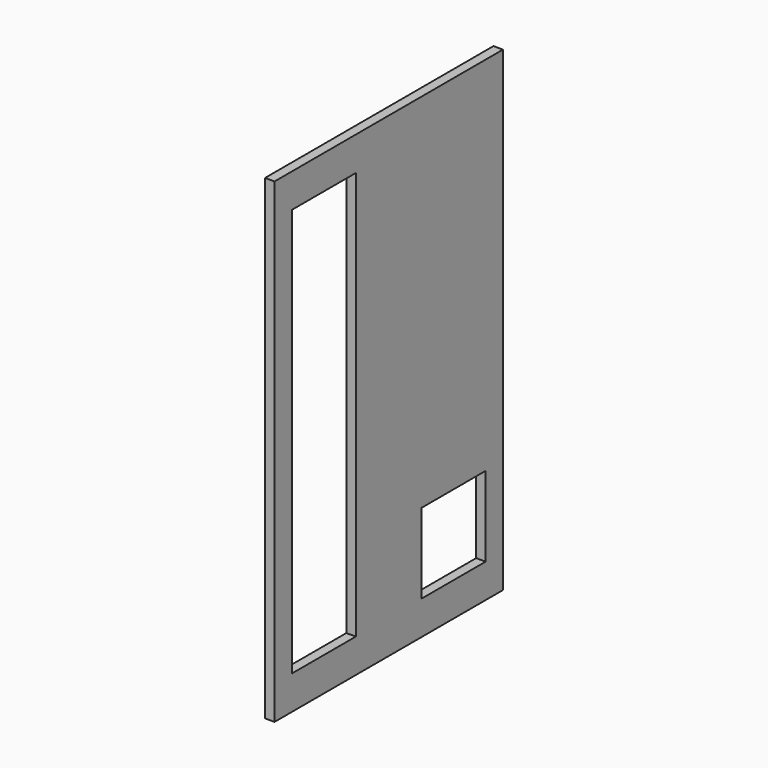
from build123d import *

# Parameters (mm, degrees)
F0_W     = 13.9900064
F0_H     = 3.81
F0_W_2   = 21
F0_H_2   = 21
F1_DEPTH = 2.5


# Not quite as in the source:
# - a feature names something its author has since deleted; it is built from what else it names


with BuildPart() as f1:
    # F0 (on Right) → F1 (new body)
    with BuildSketch(Plane.YZ):
        Polygon((4.2842663067, 140.8092032793), (4.2842663067, 15.8092032793), (79.2842663067, 15.8092032793), (79.2842663067, 140.8092032793), (75.4742663067, 140.8092032793), (75.4742663067, 136.9992032793), (75.4742663067, 19.6192032793), (8.0942663067, 19.6192032793), (8.0942663067, 136.9992032793), (55.7998448917, 136.9992032793), (61.4842599067, 136.9992032793), (61.4842599067, 140.8092032793), (55.7998448917, 140.8092032793), (11.2942599067, 140.8092032793), align=None)
        with Locations((68.4792631067, 138.9042032793)):
            Rectangle(F0_W, F0_H)
        Polygon((75.4742663067, 19.6192032793), (75.4742663067, 136.9992032793), (61.4842599067, 136.9992032793), (55.7998448917, 136.9992032793), (8.0942663067, 136.9992032793), (8.0942663067, 19.6192032793), align=None)
        Polygon((9.9742727067, 45.6992032793), (9.9742727067, 131.9192032793), (30.9742727067, 131.9192032793), (30.9742727067, 110.9192032793), (30.9742727067, 45.6992032793), (30.9742727067, 24.6992032793), (9.9742727067, 24.6992032793), align=None, mode=Mode.SUBTRACT)
        with Locations((63.0942599067, 35.1992032793)):
            Rectangle(F0_W_2, F0_H_2, mode=Mode.SUBTRACT)
    extrude(amount=F1_DEPTH)


solid = f1.part
